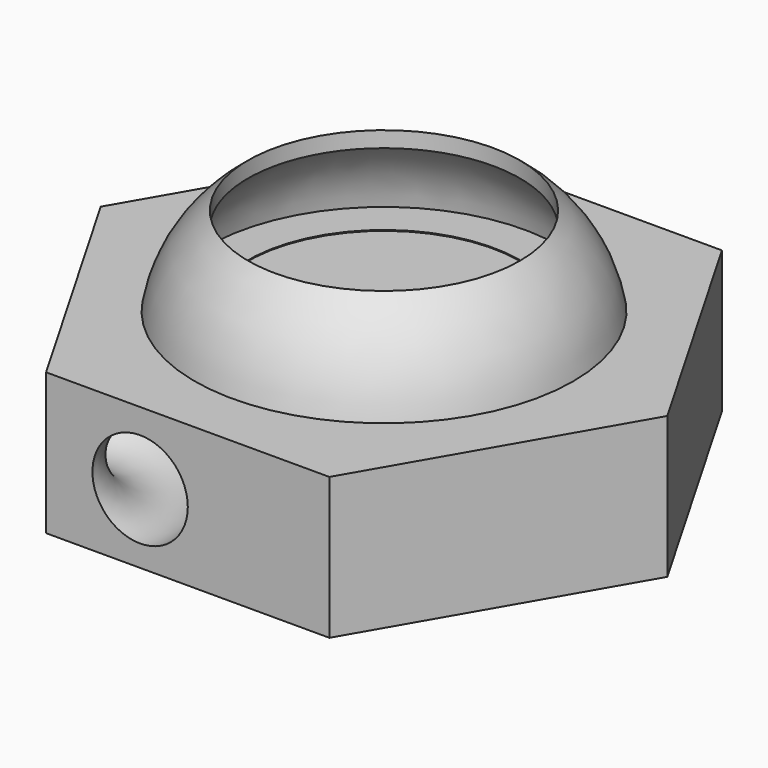
from build123d import *

# Parameters (mm, degrees)
F1_DEPTH = 7.62
F2_R     = 10.1865714181
F3_DEPTH = 6.35
F5_R     = 7.316904296
F6_DEPTH = 6.35
F9_R     = 2.5656803157


# Not quite as in the source:
# - a fillet or chamfer that OpenCascade refuses, or shapes differently, is made with other operations: its cross-section is extruded or revolved along the edge and cut away or added


with BuildPart() as f1:
    # F0 (on Top) → F1 (new body)
    with BuildSketch(Plane.XY):
        Polygon((7.62, -13.1982271537), (15.24, 0), (7.62, 13.1982271537), (-7.62, 13.1982271537), (-15.24, 0), (-7.62, -13.1982271537), align=None)
    extrude(amount=F1_DEPTH)

    # F2 (on face) → F3 (join)
    with BuildSketch(Plane.XY.offset(7.62)):
        Circle(F2_R)
    extrude(amount=F3_DEPTH)

    # F4: fillet of radius 7.62 on 1 edges, made by hand

    # F4_s1 → F4_t2 (revolve, cut)
    with BuildSketch(Plane.XZ):
        with BuildLine():
            ThreePointArc((10.1865714181, 7.62), (7.5918389432, 12.1698711326), (2.6731500935, 13.97))
            Line((2.6731500935, 13.97), (10.1865714181, 13.97))
            Line((10.1865714181, 13.97), (10.1865714181, 7.62))
        make_face()
    revolve(axis=Axis((0, 0, 13.97), (0, 0, 1)), mode=Mode.SUBTRACT)

    # F5 (on face) → F6 (cut, through all)
    with BuildSketch(Plane.XY.offset(13.97)):
        Circle(F5_R)
    extrude(amount=-F6_DEPTH, mode=Mode.SUBTRACT)

    # F7 (on Front) → F8 (revolve, cut)
    with BuildSketch(Plane.XZ):
        with BuildLine():
            Line((7.2382027283, 7.666405756), (9.4514777884, 7.6440493576))
            ThreePointArc((9.4514777884, 7.6440493576), (8.7401460246, 9.8436861794), (7.2382027283, 11.6011165082))
            Line((7.2382027283, 11.6011165082), (7.2382027283, 7.666405756))
        make_face()
    revolve(axis=Axis((0, 0, 13.97), (0, 0, 1)), mode=Mode.SUBTRACT)

    # F9 (on face) → F10 (revolve, cut)
    with BuildSketch(Plane.XZ.offset(13.1982271537)):
        with Locations((-2.5616665371, 3.7216017954)):
            Circle(F9_R)
    revolve(axis=Axis((-7.62, -13.1982271537, 3.81), (0, 0, -1)), mode=Mode.SUBTRACT)


solid = f1.part
